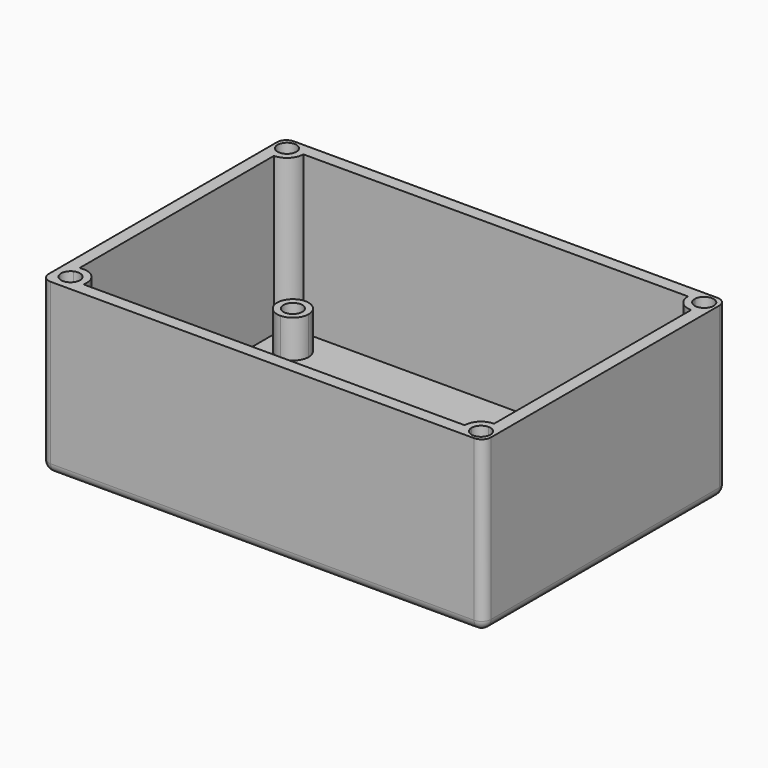
from build123d import *

# Parameters (mm, degrees)
F0_W      = 70.4
F0_H      = 48.4
F2_DEPTH  = 27
F3_T      = -2
F4_R      = 1.5
F1_R      = 2
F1_R_2    = 3.75
F5_DEPTH  = 25
F6_DEPTH  = 8
F1_W      = 35.2
F1_H      = 19.2
F7_DEPTH  = 25
F9_DEPTH  = 25
F11_DEPTH = 25


# Not quite as in the source:
# - a feature names something its author has since deleted; it is built from what else it names


with BuildPart() as f2:
    # F0 (on Top) → F2 (new body)
    with BuildSketch(Plane.XY):
        Rectangle(F0_W, F0_H)
    extrude(amount=F2_DEPTH)

    # F3
    f3_openings = [f2.faces().sort_by_distance(p)[0] for p in [
        (0, 0, 27),
    ]]
    offset(amount=F3_T, openings=f3_openings)

    # F4
    f4_edges = [f2.edges().sort_by_distance(p)[0] for p in [
        (-35.2, 24.2, 13.5),
        (-35.2, -24.2, 13.5),
        (-35.2, 0, 0),
        (0, 24.2, 0),
        (0, -24.2, 0),
        (35.2, 0, 0),
        (35.2, -24.2, 13.5),
        (35.2, 24.2, 13.5),
    ]]
    fillet(f4_edges, radius=F4_R)

    # F1 (on Top) → F5 (cut)
    with BuildSketch(Plane.XY):
        with Locations((-22.1, -13.1)):
            Circle(F1_R)
        with Locations((-22.1, 2.4)):
            Circle(F1_R_2)
    extrude(amount=F5_DEPTH, mode=Mode.SUBTRACT)

    # F1 (on Top) → F6 (join)
    with BuildSketch(Plane.XY):
        with BuildLine():
            Line((27, 17.5), (26, 17.5))
            ThreePointArc((26, 17.5), (26.732233047, 15.732233047), (28.5, 15))
            Line((28.5, 15), (28.5, 16))
            ThreePointArc((28.5, 16), (27.4393398282, 16.4393398282), (27, 17.5))
        make_face()
        with BuildLine():
            ThreePointArc((31, 17.5), (28.5, 20), (26, 17.5))
            Line((26, 17.5), (27, 17.5))
            ThreePointArc((27, 17.5), (28.5, 19), (30, 17.5))
            ThreePointArc((30, 17.5), (29.5606601718, 16.4393398282), (28.5, 16))
            Line((28.5, 16), (28.5, 15))
            ThreePointArc((28.5, 15), (30.267766953, 15.732233047), (31, 17.5))
        make_face()
        with BuildLine():
            Line((28.5, -16), (28.5, -15))
            ThreePointArc((28.5, -15), (26.732233047, -15.732233047), (26, -17.5))
            Line((26, -17.5), (27, -17.5))
            ThreePointArc((27, -17.5), (27.4393398282, -16.4393398282), (28.5, -16))
        make_face()
        with BuildLine():
            ThreePointArc((31, -17.5), (30.267766953, -15.732233047), (28.5, -15))
            Line((28.5, -15), (28.5, -16))
            ThreePointArc((28.5, -16), (29.5606601718, -16.4393398282), (30, -17.5))
            ThreePointArc((30, -17.5), (28.5, -19), (27, -17.5))
            Line((27, -17.5), (26, -17.5))
            ThreePointArc((26, -17.5), (28.5, -20), (31, -17.5))
        make_face()
        with BuildLine():
            Line((-28.5, -16), (-28.5, -15))
            ThreePointArc((-28.5, -15), (-30.267766953, -19.267766953), (-26, -17.5))
            Line((-26, -17.5), (-27, -17.5))
            ThreePointArc((-27, -17.5), (-29.5606601718, -18.5606601718), (-28.5, -16))
        make_face()
        with BuildLine():
            ThreePointArc((-26, -17.5), (-26.732233047, -15.732233047), (-28.5, -15))
            Line((-28.5, -15), (-28.5, -16))
            ThreePointArc((-28.5, -16), (-27.4393398282, -16.4393398282), (-27, -17.5))
            Line((-27, -17.5), (-26, -17.5))
        make_face()
        with BuildLine():
            Line((-27, 17.5), (-26, 17.5))
            ThreePointArc((-26, 17.5), (-30.267766953, 19.267766953), (-28.5, 15))
            Line((-28.5, 15), (-28.5, 16))
            ThreePointArc((-28.5, 16), (-29.5606601718, 18.5606601718), (-27, 17.5))
        make_face()
        with BuildLine():
            ThreePointArc((-28.5, 15), (-26.732233047, 15.732233047), (-26, 17.5))
            Line((-26, 17.5), (-27, 17.5))
            ThreePointArc((-27, 17.5), (-27.4393398282, 16.4393398282), (-28.5, 16))
            Line((-28.5, 16), (-28.5, 15))
        make_face()
    extrude(amount=F6_DEPTH)

    # F1 (on Top) → F7 (cut)
    with BuildSketch(Plane.XY):
        with Locations((8.5, 3.5)):
            Rectangle(F1_W, F1_H)
    extrude(amount=F7_DEPTH, mode=Mode.SUBTRACT)

    # F8 (on face) → F9 (join)
    with BuildSketch(Plane.XY.offset(2)):
        with BuildLine():
            ThreePointArc((-33.2, 19.6), (-31.3615223689, 20.3615223689), (-30.6, 22.2))
            Line((-30.6, 22.2), (-31.7, 22.2))
            ThreePointArc((-31.7, 22.2), (-32.1393398282, 21.1393398282), (-33.2, 20.7))
            Line((-33.2, 20.7), (-33.2, 19.6))
        make_face()
        with BuildLine():
            Line((31.7, 22.2), (30.6, 22.2))
            ThreePointArc((30.6, 22.2), (31.3615223689, 20.3615223689), (33.2, 19.6))
            Line((33.2, 19.6), (33.2, 20.7))
            ThreePointArc((33.2, 20.7), (32.1393398282, 21.1393398282), (31.7, 22.2))
        make_face()
        with BuildLine():
            Line((33.2, -20.7), (33.2, -19.6))
            ThreePointArc((33.2, -19.6), (31.3615223689, -20.3615223689), (30.6, -22.2))
            Line((30.6, -22.2), (31.7, -22.2))
            ThreePointArc((31.7, -22.2), (32.1393398282, -21.1393398282), (33.2, -20.7))
        make_face()
        with BuildLine():
            ThreePointArc((-30, -21.6), (-30.9875484503, -19.5603921946), (-33.2, -19.0701778719))
            Line((-33.2, -19.0701778719), (-33.2, -20.2252272915))
            ThreePointArc((-33.2, -20.2252272915), (-31.7784161637, -20.3450099602), (-31.1, -21.6))
            ThreePointArc((-31.1, -21.6), (-31.1316405306, -21.9064644655), (-31.2252272915, -22.2))
            Line((-31.2252272915, -22.2), (-30.0701778719, -22.2))
            ThreePointArc((-30.0701778719, -22.2), (-30.0176040647, -21.9020450851), (-30, -21.6))
        make_face()
    extrude(amount=F9_DEPTH)

    # F10 (on face) → F11 (cut)
    with BuildSketch(Plane.XY.offset(27)):
        with BuildLine():
            Line((-33.2, 22.2), (-31.7, 22.2))
            ThreePointArc((-31.7, 22.2), (-34.2606601718, 23.2606601718), (-33.2, 20.7))
            Line((-33.2, 20.7), (-33.2, 22.2))
        make_face()
        with BuildLine():
            ThreePointArc((-33.2, 20.7), (-32.1393398282, 21.1393398282), (-31.7, 22.2))
            Line((-31.7, 22.2), (-33.2, 22.2))
            Line((-33.2, 22.2), (-33.2, 20.7))
        make_face()
        with BuildLine():
            ThreePointArc((33.2, 20.7), (34.2606601718, 21.1393398282), (34.7, 22.2))
            ThreePointArc((34.7, 22.2), (33.2, 23.7), (31.7, 22.2))
            Line((31.7, 22.2), (33.2, 22.2))
            Line((33.2, 22.2), (33.2, 20.7))
        make_face()
        with BuildLine():
            Line((33.2, 22.2), (31.7, 22.2))
            ThreePointArc((31.7, 22.2), (32.1393398282, 21.1393398282), (33.2, 20.7))
            Line((33.2, 20.7), (33.2, 22.2))
        make_face()
        with BuildLine():
            ThreePointArc((31.7, -22.2), (33.2, -23.7), (34.7, -22.2))
            ThreePointArc((34.7, -22.2), (34.2606601718, -21.1393398282), (33.2, -20.7))
            Line((33.2, -20.7), (33.2, -22.2))
            Line((33.2, -22.2), (31.7, -22.2))
        make_face()
        with BuildLine():
            Line((-33.2, -22.2), (-33.2, -20.2252272915))
            ThreePointArc((-33.2, -20.2252272915), (-33.6606601718, -22.6606601718), (-31.2252272915, -22.2))
            Line((-31.2252272915, -22.2), (-33.2, -22.2))
        make_face()
    extrude(amount=-F11_DEPTH, mode=Mode.SUBTRACT)


solid = f2.part
